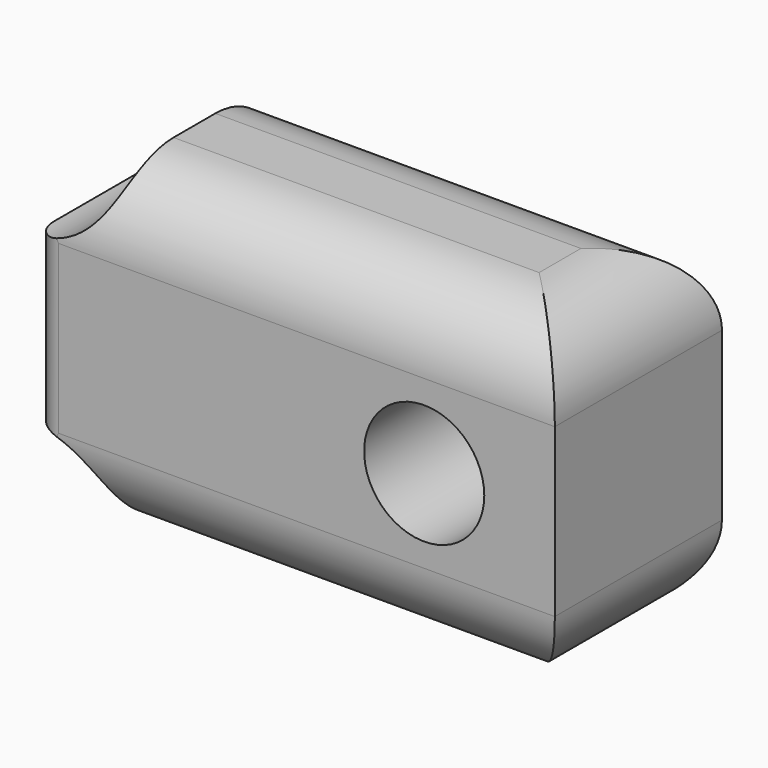
from build123d import *

# Parameters (mm, degrees)
F0_R     = 1.15
F1_DEPTH = 4
F2_R     = 1.5
F3_DEPTH = 5
F4_R     = 1.5
F5_R     = 0.49999


# Not quite as in the source:
# - a fillet or chamfer is up to 0.001 mm smaller than in the source, because OpenCascade refuses the exact size


with BuildPart() as f1:
    # F0 (on Front) → F1 (new body)
    with BuildSketch(Plane.XZ):
        with BuildLine():
            Line((5, 3.1), (-3.5, 3.1))
            ThreePointArc((-3.5, 3.1), (-3.93934, 2.03934), (-5, 1.6))
            Line((-5, 1.6), (-5, -1.6))
            ThreePointArc((-5, -1.6), (-3.93934, -2.03934), (-3.5, -3.1))
            Line((-3.5, -3.1), (5, -3.1))
            Line((5, -3.1), (5, 3.1))
        make_face()
        with Locations((2.5, 0)):
            Circle(F0_R, mode=Mode.SUBTRACT)
    extrude(amount=F1_DEPTH)

    # F2 (on face) → F3 (cut)
    with BuildSketch(Plane(origin=(-5, 0, 0), x_dir=(0, -1, 0), z_dir=(-1, 0, 0))):
        with Locations((2, 0)):
            Circle(F2_R)
    extrude(amount=-F3_DEPTH, mode=Mode.SUBTRACT)

    # F4
    f4_edges = [f1.edges().sort_by_distance(p)[0] for p in [
        (0.75, -4, 3.1),
        (0.75, 0, 3.1),
        (0.75, -4, -3.1),
        (0.75, 0, -3.1),
        (5, -2, 3.1),
        (5, -2, -3.1),
    ]]
    fillet(f4_edges, radius=F4_R)

    # F5 (radius 0.5 in the source; OpenCascade refuses exactly that, so slightly less here)
    f5_edges = [f1.edges().sort_by_distance(p)[0] for p in [
        (-5, -4, 0),
        (-5, 0, 0),
    ]]
    fillet(f5_edges, radius=F5_R)


solid = f1.part
